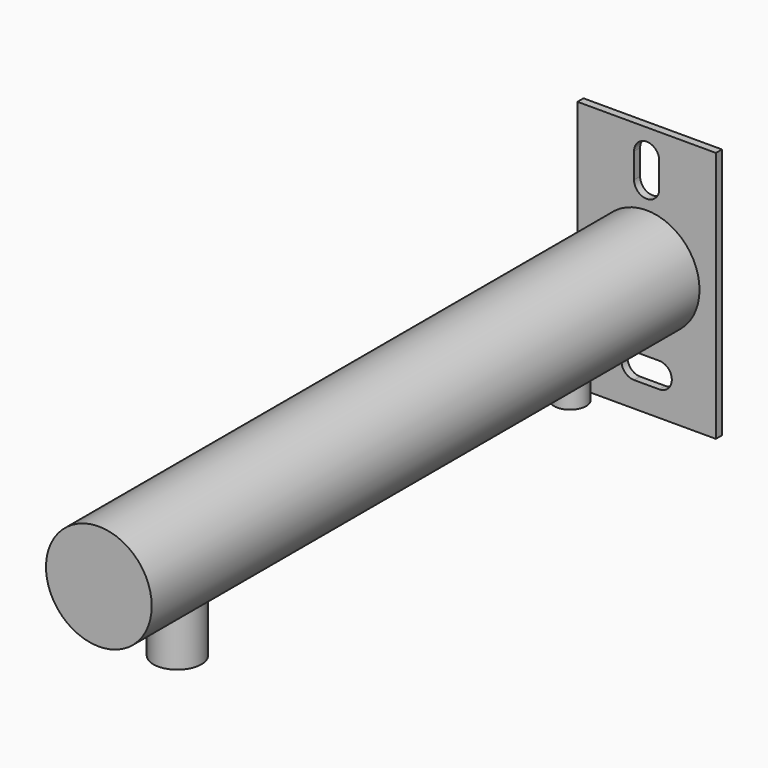
from build123d import *

# Parameters (mm, degrees)
F0_W     = 55
F0_H     = 100
F1_DEPTH = 3
F2_R     = 21
F3_DEPTH = 272
F4_R     = 6.35
F5_DEPTH = 30
F4_R_2   = 9.525
F6_DEPTH = 40


# Not quite as in the source:
# - a feature names something its author has since deleted; it is built from what else it names


with BuildPart() as f1:
    # F0 (on Front) → F1 (new body)
    with BuildSketch(Plane.XZ):
        Rectangle(F0_W, F0_H)
        with BuildLine():
            ThreePointArc((-10, -35), (-8.5355339059, -31.4644660941), (-5, -30))
            Line((-5, -30), (0, -30))
            Line((0, -30), (5, -30))
            ThreePointArc((5, -30), (8.5355339059, -31.4644660941), (10, -35))
            ThreePointArc((10, -35), (8.5355339059, -38.5355339059), (5, -40))
            Line((5, -40), (0, -40))
            Line((0, -40), (-5, -40))
            ThreePointArc((-5, -40), (-8.5355339059, -38.5355339059), (-10, -35))
        make_face(mode=Mode.SUBTRACT)
        with BuildLine():
            Line((-5, 30), (-5, 40))
            ThreePointArc((-5, 40), (0, 45), (5, 40))
            Line((5, 40), (5, 30))
            ThreePointArc((5, 30), (0, 25), (-5, 30))
        make_face(mode=Mode.SUBTRACT)
    extrude(amount=F1_DEPTH)

    # F2 (on face) → F3 (join)
    with BuildSketch(Plane.XZ.offset(3)):
        Circle(F2_R)
    extrude(amount=F3_DEPTH)

    # F4 (on Top) → F5 (join)
    with BuildSketch(Plane.XY):
        with Locations((0, -41)):
            Circle(F4_R)
    extrude(amount=-F5_DEPTH)

    # F4 (on Top) → F6 (join)
    with BuildSketch(Plane.XY):
        with Locations((0, -236)):
            Circle(F4_R_2)
    extrude(amount=-F6_DEPTH)


solid = f1.part
